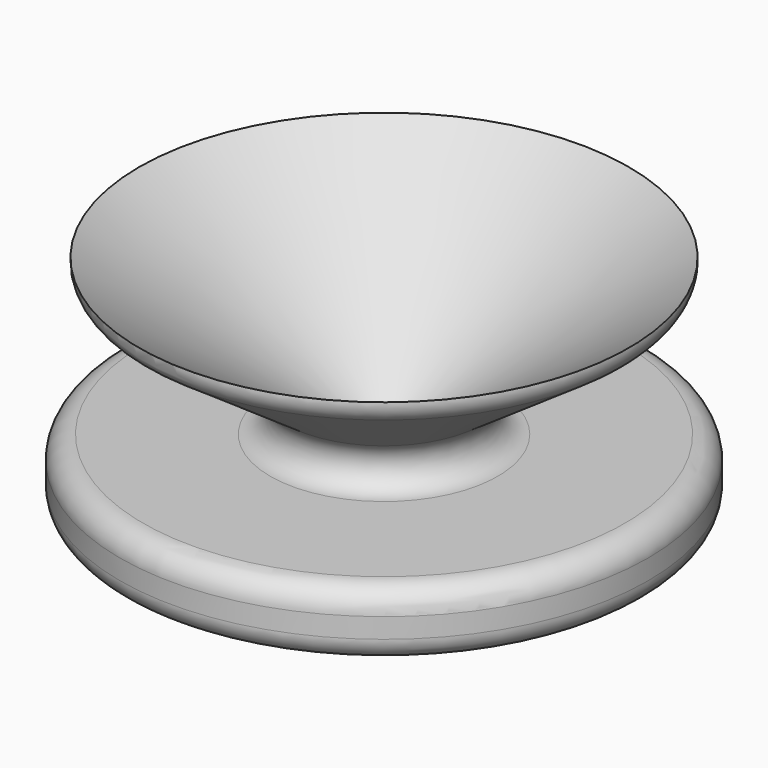
from build123d import *

# Parameters (mm, degrees)
F2_T = -2.54


# Not quite as in the source:
# - a fillet or chamfer that OpenCascade refuses, or shapes differently, is made with other operations: its cross-section is extruded or revolved along the edge and cut away or added


with BuildPart() as f1:
    # F0 (on Front) → F1 (revolve)
    with BuildSketch(Plane.XZ):
        Polygon((-8.6911804974, 13.8674174355), (0, 13.8674174355), (0, 48.0571240187), (-58.2820437849, 48.0571240187), align=None)
        Polygon((-58.0264218152, 0), (0, 0), (0, 13.8674174355), (-8.6911804974, 13.8674174355), (-58.0264218152, 13.8674174355), align=None)
    revolve(axis=Axis((0, 0, 30.9622707271), (0, 0, -1)))

    # F2
    f2_openings = [f1.faces().sort_by_distance(p)[0] for p in [
        (0, 0, 48.057124),
        (0, 0, 0),
    ]]
    offset(amount=F2_T, openings=f2_openings, kind=Kind.INTERSECTION)

    # F3: fillet of radius 5.08 on 6 edges, made by hand

    # F3_s1 → F3_t2 (revolve)
    with BuildSketch(Plane.XZ):
        with BuildLine():
            ThreePointArc((-22.1258654795, 23.1297675365), (-20.1589276546, 17.4374403683), (-25.0093265306, 13.8674174355))
            Line((-25.0093265306, 13.8674174355), (-8.6911804974, 13.8674174355))
            Line((-8.6911804974, 13.8674174355), (-22.1258654795, 23.1297675365))
        make_face()
    revolve(axis=Axis((0, 0, 13.8674174355), (0, 0, -1)))

    # F3_s3 → F3_t4 (revolve, cut)
    with BuildSketch(Plane.XZ):
        with BuildLine():
            ThreePointArc((-51.6268528261, 43.4687984471), (-53.3317173465, 45.4708576387), (-53.8071437354, 48.0571240187))
            Line((-53.8071437354, 48.0571240187), (-58.2820437849, 48.0571240187))
            Line((-58.2820437849, 48.0571240187), (-51.6268528261, 43.4687984471))
        make_face()
    revolve(axis=Axis((0, 0, 48.0571240187), (0, 0, -1)), mode=Mode.SUBTRACT)

    # F3_s5 → F3_t6 (revolve, cut)
    with BuildSketch(Plane.XZ):
        with BuildLine():
            ThreePointArc((-52.9464218152, 13.8674174355), (-56.5385242636, 12.3795198839), (-58.0264218152, 8.7874174355))
            Line((-58.0264218152, 8.7874174355), (-58.0264218152, 13.8674174355))
            Line((-58.0264218152, 13.8674174355), (-52.9464218152, 13.8674174355))
        make_face()
    revolve(axis=Axis((0, 0, 13.8674174355), (0, 0, -1)), mode=Mode.SUBTRACT)

    # F3_s7 → F3_t8 (revolve, cut)
    with BuildSketch(Plane.XZ):
        with BuildLine():
            ThreePointArc((-58.0264218152, 4.3994090512), (-57.3458308664, 1.8594090512), (-55.4864218152, 0))
            Line((-55.4864218152, 0), (-58.0264218152, 0))
            Line((-58.0264218152, 0), (-58.0264218152, 4.3994090512))
        make_face()
    revolve(axis=Axis((0, 0, 0), (0, 0, -1)), mode=Mode.SUBTRACT)


solid = f1.part
